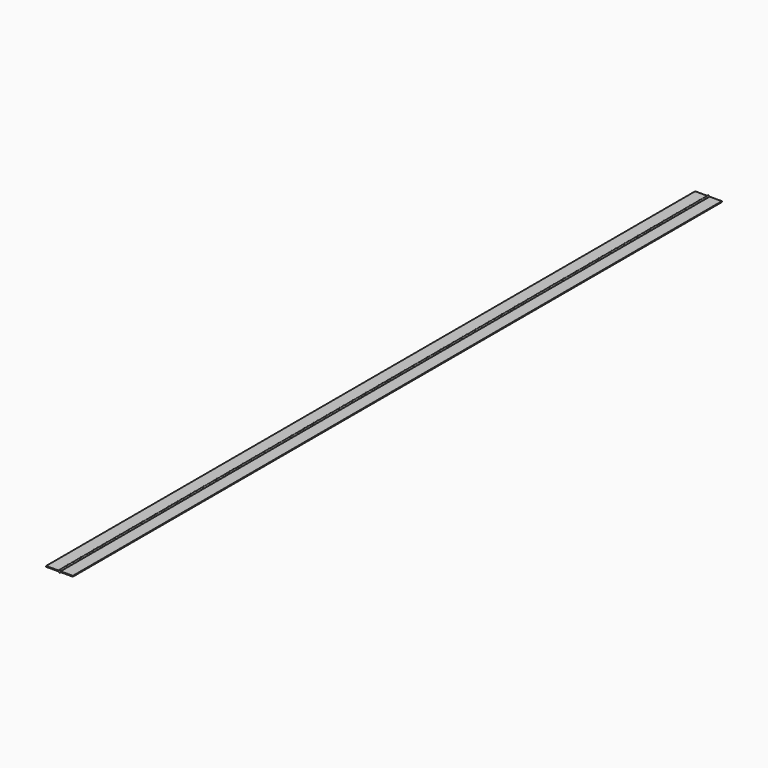
from build123d import *

# Parameters (mm, degrees)
F0_R     = 1.5
F1_DEPTH = 500
F2_W     = 16.5
F2_H     = 1
F3_DEPTH = 500
F4_R     = 1.5
F5_DEPTH = 500
F6_W     = 16.5
F6_H     = 1
F7_DEPTH = 500


with BuildPart() as f1:
    # F0 (on Front) → F1 (new body, symmetric)
    with BuildSketch(Plane.XZ):
        Circle(F0_R)
    extrude(amount=F1_DEPTH, both=True)

    # F2 (on Front) → F3 (join, symmetric)
    with BuildSketch(Plane.XZ):
        with Locations((8.25, 0)):
            Rectangle(F2_W, F2_H)
    extrude(amount=F3_DEPTH, both=True)


with BuildPart() as f5:
    # F4 (on Front) → F5 (new body, symmetric)
    with BuildSketch(Plane.XZ):
        Circle(F4_R)
    extrude(amount=F5_DEPTH, both=True)

    # F6 (on Front) → F7 (join, symmetric)
    with BuildSketch(Plane.XZ):
        with Locations((-8.25, 0)):
            Rectangle(F6_W, F6_H)
    extrude(amount=F7_DEPTH, both=True)


solid = Compound([f1.part, f5.part])
